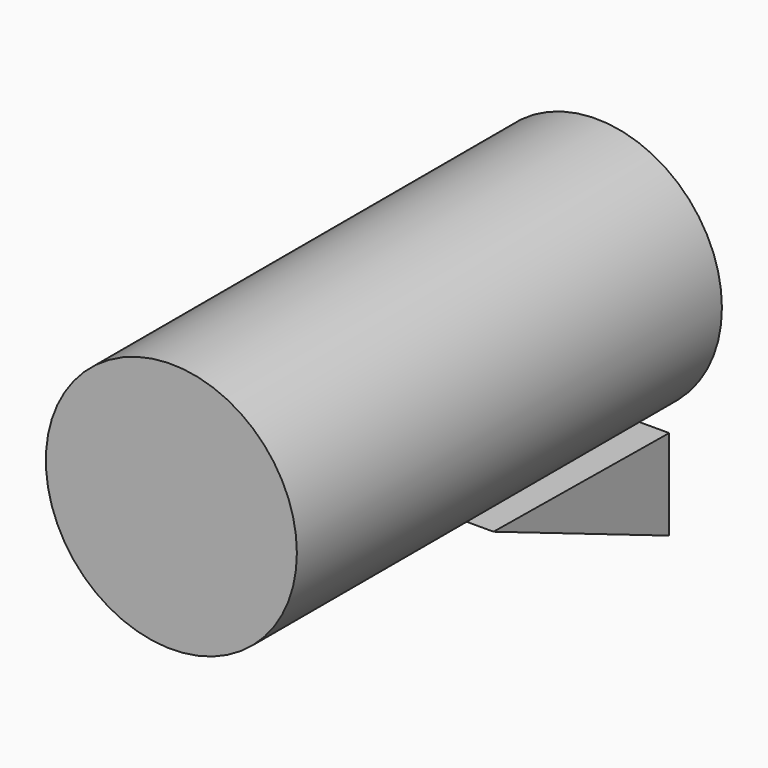
from build123d import *

# Parameters (mm, degrees)
F0_R     = 43.8070462956
F1_DEPTH = 90.678
F2_DEPTH = 94.742
F7_DEPTH = 25.4


# Not quite as in the source:
# - the program builds the solid bodies; features that only make, move or delete a surface that nothing else refers to are left out


with BuildPart() as f1:
    # F0 (on Front) → F1 (new body)
    with BuildSketch(Plane.XZ):
        Circle(F0_R)
    extrude(amount=F1_DEPTH)

    # F2 (add): a face of the model
    f2_faces = [f1.faces().sort_by_distance(p)[0] for p in [
        (0, -90.678, 0),
    ]]
    extrude(f2_faces, amount=F2_DEPTH)

    # F4 (on Right) → F7 (join)
    with BuildSketch(Plane.YZ):
        Polygon((0, -44.503852725), (-76.628126204, -43.6692126095), (0, -76.0243907571), align=None)
    extrude(amount=F7_DEPTH)


solid = f1.part
